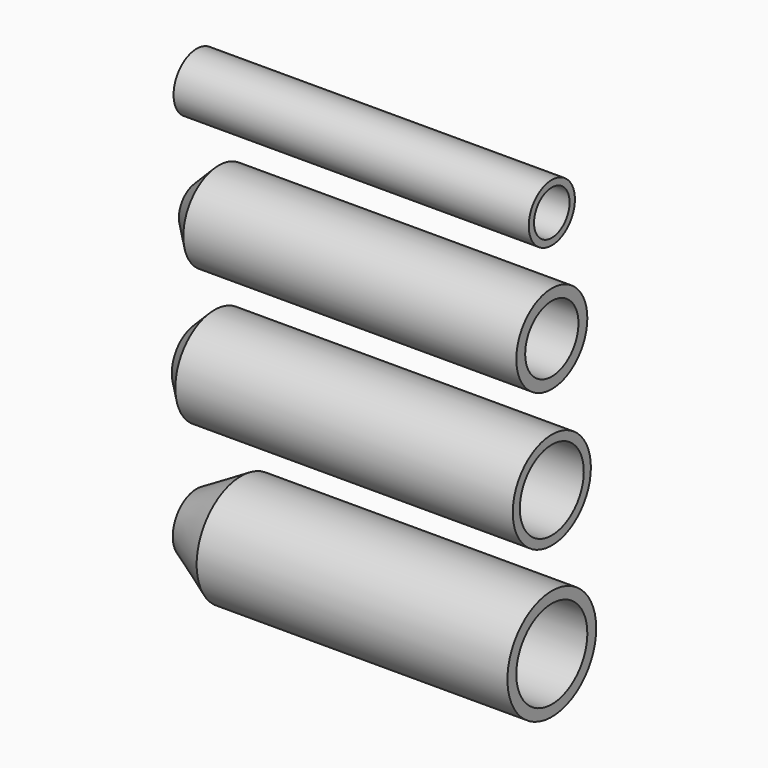
from build123d import *

# Parameters (mm, degrees)
F0_R     = 1.1
F1_DEPTH = 4
F0_R_2   = 1
F0_R_3   = 1.25
F0_R_4   = 0.65
F3_D     = 1
F4_D     = 1.3
F5_D     = 1.4
F6_D     = 1
F7_SIZE2 = 0.39999
F7_SIZE  = 0.39999
F8_SIZE2 = 0.49999
F8_SIZE  = 0.49999
F9_SIZE2 = 0.5773502692
F9_SIZE  = 1


# Not quite as in the source:
# - a fillet or chamfer is up to 0.001 mm smaller than in the source, because OpenCascade refuses the exact size


with BuildPart() as f1:
    # F0 (on Right) → F1 (new body, symmetric)
    with BuildSketch(Plane.YZ):
        Circle(F0_R)
    extrude(amount=F1_DEPTH, both=True)

    # F5 (through all)
    with Locations(Plane.YZ.offset(4)):
        with Locations((0, 0)):
            Hole(F5_D / 2)

    # F7 (size 0.4 and 0.4 in the source; OpenCascade refuses exactly that, so slightly less here)
    f7_edges = [f1.edges().sort_by_distance(p)[0] for p in [
        (-4, -1.1, 0),
    ]]
    chamfer(f7_edges, length=F7_SIZE, length2=F7_SIZE2)

    # F12 (on Front) → F13 (revolve, cut)
    with BuildSketch(Plane.XZ):
        Polygon((0, 0.7), (0, 0), (4, 0), (4, 0.9), (0.2, 0.9), align=None)
    revolve(axis=Axis((2, 0, 0), (1, 0, 0)), mode=Mode.SUBTRACT)


with BuildPart() as f1b:
    # F0 (on Right) → F1, piece 2 (new body, symmetric)
    with BuildSketch(Plane.YZ):
        with Locations((0, 3)):
            Circle(F0_R_2)
    extrude(amount=F1_DEPTH, both=True)

    # F6 (through all)
    with Locations(Plane.YZ.offset(4)):
        with Locations((0, 3)):
            Hole(F6_D / 2)

    # F8 (size 0.5 and 0.5 in the source; OpenCascade refuses exactly that, so slightly less here)
    f8_edges = [f1b.edges().sort_by_distance(p)[0] for p in [
        (-4, -1, 3),
    ]]
    chamfer(f8_edges, length=F8_SIZE, length2=F8_SIZE2)

    # F14 (on Front) → F15 (revolve, cut)
    with BuildSketch(Plane.XZ):
        Polygon((0, 3), (4, 3), (4, 3.75), (0.25, 3.75), (0, 3.5), align=None)
    revolve(axis=Axis((2, 0, 3), (-1, 0, 0)), mode=Mode.SUBTRACT)


with BuildPart() as f1c:
    # F0 (on Right) → F1, piece 3 (new body, symmetric)
    with BuildSketch(Plane.YZ):
        with Locations((0, -3.25)):
            Circle(F0_R_3)
    extrude(amount=F1_DEPTH, both=True)

    # F4 (through all)
    with Locations(Plane.YZ.offset(4)):
        with Locations((0, -3.25)):
            Hole(F4_D / 2)

    # F9
    f9_edges = [f1c.edges().sort_by_distance(p)[0] for p in [
        (-4, -1.25, -3.25),
    ]]
    f9_side = f1c.faces().sort_by_distance((0, -1.25, -3.25))[0]
    chamfer(f9_edges, length=F9_SIZE, length2=F9_SIZE2, reference=f9_side)

    # F10 (on Front) → F11 (revolve, cut)
    with BuildSketch(Plane.XZ):
        Polygon((4, -3.25), (4, -2.25), (0.35, -2.25), (0, -2.6), (0, -3.25), align=None)
    revolve(axis=Axis((2, 0, -3.25), (-1, 0, 0)), mode=Mode.SUBTRACT)


with BuildPart() as f1d:
    # F0 (on Right) → F1, piece 4 (new body, symmetric)
    with BuildSketch(Plane.YZ):
        with Locations((0, 5.5)):
            Circle(F0_R_4)
    extrude(amount=F1_DEPTH, both=True)

    # F3 (through all)
    with Locations(Plane.YZ.offset(4)):
        with Locations((0, 5.5)):
            Hole(F3_D / 2)


solid = Compound([f1.part, f1b.part, f1c.part, f1d.part])
